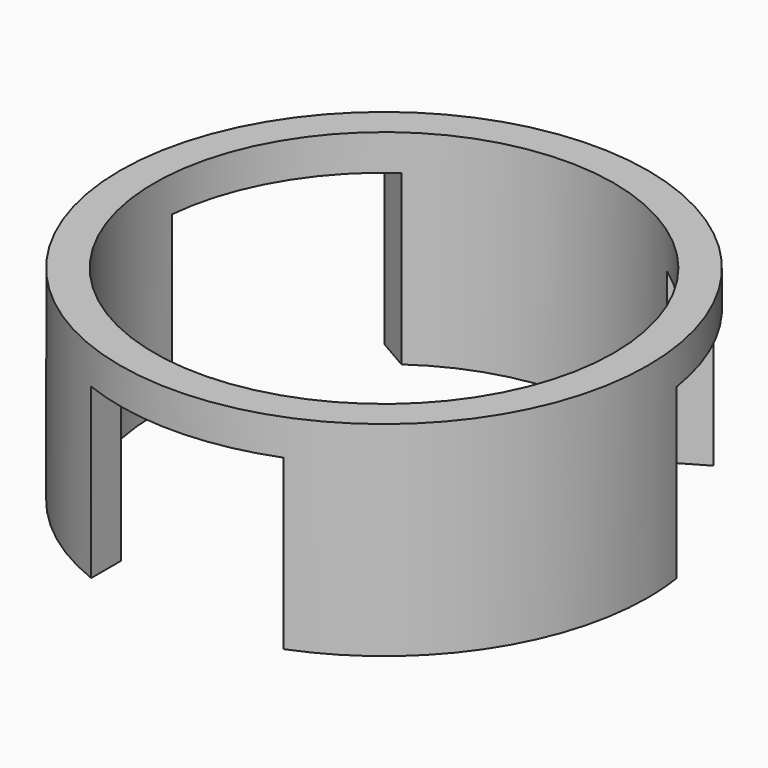
from build123d import *

# Parameters (mm, degrees)
F0_R      = 15.5
F0_R_2    = 13.5
F1_DEPTH  = 10
F3_R      = 15.5
F3_R_2    = 13.5
F4_DEPTH  = 2
F5_W      = 11.3
F5_H      = 18.3407559019
F6_DEPTH  = 9.9
F7_COUNT  = 3
F9_R      = 8
F10_DEPTH = 25


# Not quite as in the source:
# - the program builds the solid bodies; features that only make, move or delete a surface that nothing else refers to are left out


with BuildPart() as f1:
    # F0 (on Top) → F1 (new body)
    with BuildSketch(Plane.XY):
        Circle(F0_R)
        Circle(F0_R_2, mode=Mode.SUBTRACT)
    extrude(amount=F1_DEPTH)

    # F3 (on offset) → F4 (join)
    with BuildSketch(Plane.XY.offset(10)):
        Circle(F3_R)
        Circle(F3_R_2, mode=Mode.SUBTRACT)
    extrude(amount=F4_DEPTH)

    # F5 (on Top) → F6 (cut)
    with BuildSketch(Plane.XY):
        with Locations((-1.81e-07, -13.0000018069)):
            Rectangle(F5_W, F5_H)
    f6 = extrude(amount=F6_DEPTH, mode=Mode.SUBTRACT)

    # F7: F6 ×3 about axis
    f7_axis = Axis((0, 0, 0), (0, 0, -1))
    for i in range(1, F7_COUNT):
        add(f6.rotate(f7_axis, i * 360 / F7_COUNT), mode=Mode.SUBTRACT)

    # F9 (on offset) → F10 (cut)
    with BuildSketch(Plane.XY.offset(22)):
        Circle(F9_R)
    extrude(amount=-F10_DEPTH, mode=Mode.SUBTRACT)


solid = f1.part
